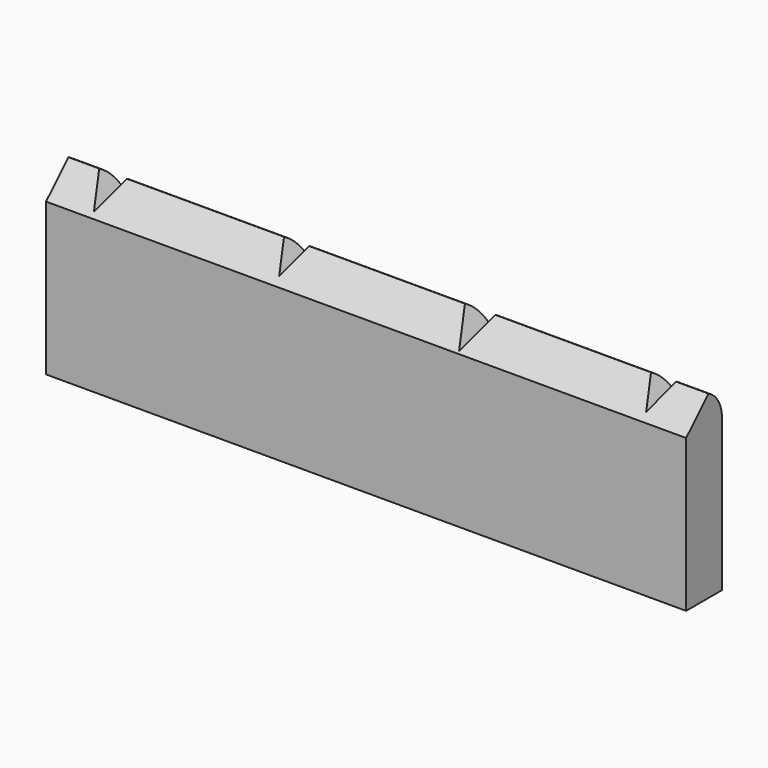
from build123d import *

# Parameters (mm, degrees)
F0_W        = 36.322
F0_H        = 2.54
F1_DEPTH    = 10.414
F3_R        = 1.778
F4_T1_DEPTH = 45.4669047052
F5_DEPTH    = 25.4


# Not quite as in the source:
# - a fillet or chamfer that OpenCascade refuses, or shapes differently, is made with other operations: its cross-section is extruded or revolved along the edge and cut away or added


with BuildPart() as f1:
    # F0 (on Top) → F1 (new body)
    with BuildSketch(Plane.XY):
        with Locations((0, 1.27)):
            Rectangle(F0_W, F0_H)
    extrude(amount=F1_DEPTH)

    # F3
    f3_edges = [f1.edges().sort_by_distance(p)[0] for p in [
        (0, 2.54, 10.414),
    ]]
    fillet(f3_edges, radius=F3_R)

    # F4: chamfer of 1.778 on 1 edges, made by hand

    # F4_s2 → F4_t1 (cut)
    with BuildSketch(Plane.YZ.offset(-22.7334523526)):
        Polygon((1.778, 10.414), (0, 8.636), (0, 10.414), align=None)
    extrude(amount=F4_T1_DEPTH, mode=Mode.SUBTRACT)

    # F2 (on face) → F5 (cut)
    with BuildSketch(Plane.XZ):
        Polygon((-15.621, 8.8492954744), (-14.7176174209, 10.414), (-16.5243825791, 10.414), align=None)
        Polygon((-4.3769409051, 10.414), (-6.0370590949, 10.414), (-5.207, 8.9762954744), align=None)
        Polygon((6.1837060633, 10.414), (4.2302939367, 10.414), (5.207, 8.7222954744), align=None)
        Polygon((16.4510590949, 10.414), (14.7909409051, 10.414), (15.621, 8.9762954744), align=None)
    extrude(amount=-F5_DEPTH, mode=Mode.SUBTRACT)


solid = f1.part
